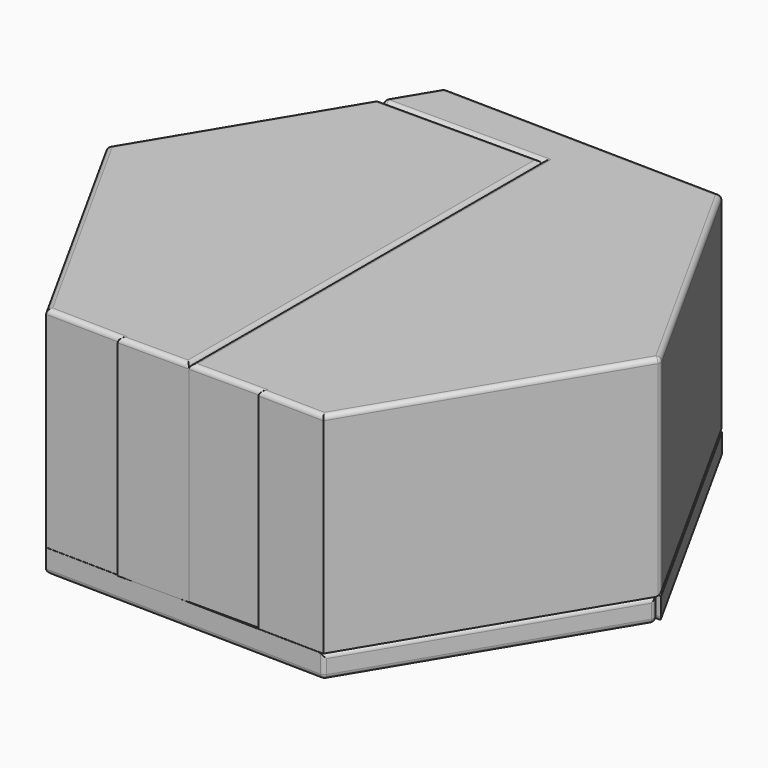
from build123d import *

# Parameters (mm, degrees)
F2_DEPTH      = 25.4
F4_DEPTH      = 76.2
F4_DEPTH_BACK = 76.2
F6_DEPTH      = 76.454
F8_DEPTH      = 227.1522
F10_DEPTH     = 25.4
F12_W         = 478.5499326668
F12_H         = 227.3464668878
F13_DEPTH     = 77.216
F15_DEPTH     = 227.3464668878
F16_W         = 76.454
F16_H         = 60.1742118597
F17_DEPTH     = 163.7678072
F18_R         = 5.08
F18_2_R       = 5.08
F20_R         = 5.08


# Not quite as in the source:
# - an extrude ends at something that could not be found from the text; its depth is read off the source's solid


with BuildPart() as f2:
    # F1 (on face) → F2 (new body)
    with BuildSketch(Plane.XY):
        Polygon((304.8, -5.5580618585), (0, 0), (-157.2134227653, -261.1855121443), (147.5865772347, -266.7435740027), align=None)
    extrude(amount=F2_DEPTH)



with BuildPart() as f4:
    # F3 (on Right) → F4 (new body, two sides)
    with BuildSketch(Plane.YZ) as f4_sk:
        Polygon((34.925, 184.9217274444), (-34.925, 184.9217274444), (-69.85, 124.4298529901), (-34.925, 63.9379785357), (34.925, 63.9379785357), (69.85, 124.4298529901), align=None)
    extrude(amount=F4_DEPTH)
    extrude(f4_sk.sketch, amount=-F4_DEPTH_BACK)

    # F20
    f20_edges = [f4.edges().sort_by_distance(p)[0] for p in [
        (76.2, 0, 184.921727),
        (0, -34.925, 184.921727),
        (-76.2, 0, 184.921727),
        (0, 34.925, 184.921727),
        (-76.2, 52.3875, 154.67579),
        (-76.2, -52.3875, 154.67579),
        (-76.2, -52.3875, 94.183916),
        (-76.2, 0, 63.937979),
        (-76.2, 52.3875, 94.183916),
        (76.2, -52.3875, 154.67579),
        (0, -69.85, 124.429853),
        (0, 69.85, 124.429853),
        (76.2, 52.3875, 154.67579),
        (76.2, -52.3875, 94.183916),
        (0, -34.925, 63.937979),
        (0, 34.925, 63.937979),
        (76.2, 52.3875, 94.183916),
    ]]
    fillet(f20_edges, radius=F20_R)


with BuildPart() as f6:
    # F5 (on Right) → F6 (new body)
    with BuildSketch(Plane.YZ):
        Polygon((-264.0685473475, 88.9786597022), (-264.0685473475, 25.8405029335), (0.254, 25.8405029335), (0.254, 0), (214.9657905102, 0), (214.9657905102, 252.7464668878), (-203.8943354878, 252.7464668878), (-203.8943354878, 88.9786597022), align=None)
        Polygon((-35.052, 185.1757274444), (35.052, 185.1757274444), (70.104, 124.4638825375), (35.052, 63.7520376306), (-35.052, 63.7520376306), (-70.104, 124.4638825375), align=None, mode=Mode.SUBTRACT)
    extrude(amount=F6_DEPTH)

    # F7 (on face) → F8 (join)
    with BuildSketch(Plane.XY.offset(252.7464668878)):
        Polygon((-178.7527874094, 214.9657905102), (0, 214.9657905102), (76.454, 214.9657905102), (76.454, -203.8943354878), (76.454, -265.4464635552), (147.5865772347, -266.7435740027), (304.8, -5.5580618585), (157.2134227653, 261.1855121443), (-147.5865772347, 266.7435740027), align=None)
    extrude(amount=-F8_DEPTH)

    # F16 (on face) → F17 (join, through all)
    with BuildSketch(Plane.XY.offset(88.9786597022)):
        with Locations((38.227, -233.9814414177)):
            Rectangle(F16_W, F16_H)
    extrude(amount=F17_DEPTH)

    # F18#2
    f18_2_edges = [f6.edges().sort_by_distance(p)[0] for p in [
        (157.213423, 261.185512, 139.170367),
        (-147.586577, 266.743574, 139.170367),
        (4.813423, 263.964543, 252.746467),
        (4.813423, 263.964543, 25.594267),
        (-178.752787, 214.965791, 139.170367),
        (-163.169682, 240.854682, 252.746467),
        (-163.169682, 240.854682, 25.594267),
        (0, -233.981441, 252.746467),
        (38.227, -264.068547, 252.746467),
        (76.454, -264.757505, 252.746467),
        (112.020289, -266.095019, 252.746467),
        (226.193289, -136.150818, 252.746467),
        (231.006711, 127.813725, 252.746467),
        (-89.376394, 214.965791, 252.746467),
        (0, 5.535728, 252.746467),
        (304.8, -5.558062, 139.170367),
        (231.006711, 127.813725, 25.594267),
    ]]
    fillet(f18_2_edges, radius=F18_2_R)


with BuildPart() as f10:
    # F9 (on face) → F10 (new body, through all)
    with BuildSketch(Plane.XY.offset(25.4)):
        Polygon((-304.8, 5.5580618585), (-157.3363911366, -260.9632627806), (-0.254, 0), (-0.254, 215.2197905102), (76.708, 215.2197905102), (76.708, 0), (304.7919404066, -5.54349519), (157.2134227653, 261.1855121443), (-147.5865772347, 266.7435740027), align=None)
    extrude(amount=-F10_DEPTH)


with BuildPart() as f2_1:
    add(f2.part)

    add(f10.part)  # F13 merges F10
    # F12 (on offset) → F13 (join)
    with BuildSketch(Plane(origin=(-0.254, 0, 0), x_dir=(0, -1, 0), z_dir=(-1, 0, 0))):
        with Locations((24.5631758232, 139.0732334439)):
            Rectangle(F12_W, F12_H)
        Polygon((-70.104, 124.4638825375), (-35.052, 185.1757274444), (35.052, 185.1757274444), (70.104, 124.4638825375), (35.052, 63.7520376306), (-35.052, 63.7520376306), align=None, mode=Mode.SUBTRACT)
    extrude(amount=F13_DEPTH)

    # F14 (on face) → F15 (join, through all)
    with BuildSketch(Plane.XY.offset(25.4)):
        Polygon((-178.9056757111, 214.7117905102), (-304.8, 5.5580618585), (-157.3363911366, -260.9632627806), (-77.216, -262.4242670131), (-77.216, 214.7117905102), align=None)
    extrude(amount=F15_DEPTH)

    # F18
    f18_edges = [f2_1.edges().sort_by_distance(p)[0] for p in [
        (-89.579838, 214.711791, 252.746467),
        (-241.852838, 110.134926, 252.746467),
        (-231.068196, -127.7026, 252.746467),
        (-117.403196, -261.691449, 252.746467),
        (-77.47, -263.128889, 252.746467),
        (-38.862, -263.838142, 252.746467),
        (-0.254, -24.563176, 252.746467),
        (-147.586577, 266.743574, 12.7),
        (-226.193289, 136.150818, 0),
        (-304.8, 5.558062, 126.373233),
        (-178.905676, 214.711791, 139.073233),
        (-163.246126, 240.727682, 25.4),
        (-231.068196, -127.7026, 0),
        (-78.795196, -130.481631, 0),
        (-0.254, 107.609895, 0),
        (38.227, 215.219791, 0),
        (76.708, 107.609895, 0),
        (190.74997, -2.771748, 0),
        (231.002682, 127.821008, 0),
        (4.813423, 263.964543, 0),
        (-4.813423, -263.964543, 0),
        (226.193289, -136.150818, 0),
        (152.4, -2.779031, 0),
        (-78.606711, -130.592756, 0),
        (147.586577, -266.743574, 12.7),
        (304.8, -5.558062, 12.7),
        (226.193289, -136.150818, 25.4),
    ]]
    fillet(f18_edges, radius=F18_R)


solid = Compound([f4.part, f6.part, f2_1.part])
